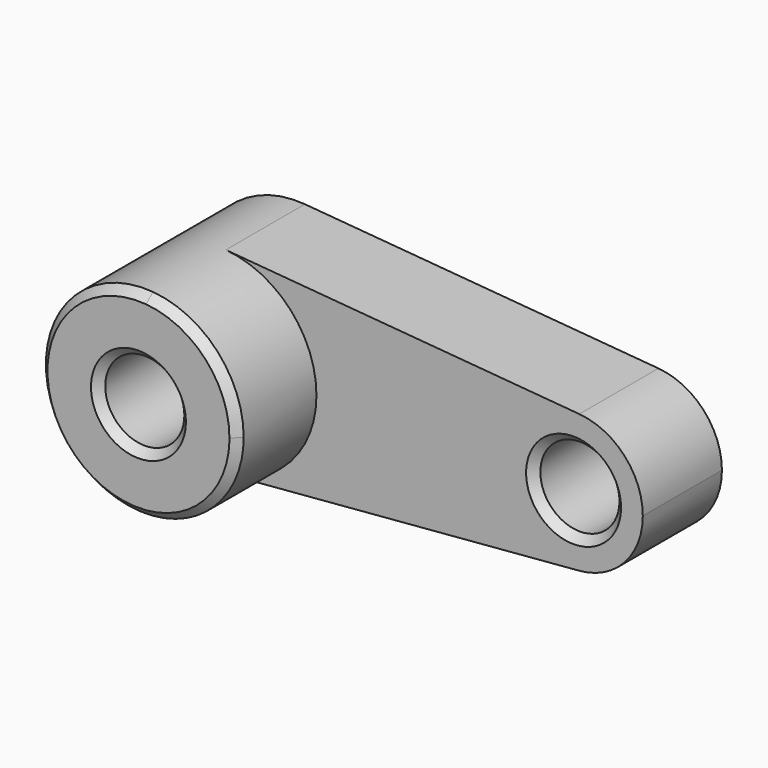
from build123d import *

# Parameters (mm, degrees)
F0_R     = 10
F1_DEPTH = 25
F2_DEPTH = 50
F3_SIZE  = 2


# Not quite as in the source:
# - the program builds the solid bodies; features that only make, move or delete a surface that nothing else refers to are left out


with BuildPart() as f1:
    # F0 (on Front) → F1 (new body)
    with BuildSketch(Plane.XZ):
        with BuildLine():
            ThreePointArc((2.0833333333, -24.9130432148), (18.3995018048, -16.9250800097), (25, 0))
            ThreePointArc((25, 0), (18.3995018048, 16.9250800097), (2.0833333333, 24.9130432148))
            ThreePointArc((2.0833333333, 24.9130432148), (-25, 0), (2.0833333333, -24.9130432148))
        make_face()
        Circle(F0_R, mode=Mode.SUBTRACT)
        with BuildLine():
            ThreePointArc((2.0833333333, 24.9130432148), (18.3995018048, 16.9250800097), (25, 0))
            ThreePointArc((25, 0), (18.3995018048, -16.9250800097), (2.0833333333, -24.9130432148))
            Line((2.0833333333, -24.9130432148), (91.4583333333, -17.4391302504))
            ThreePointArc((91.4583333333, -17.4391302504), (72.5, 0), (91.4583333333, 17.4391302504))
            Line((91.4583333333, 17.4391302504), (2.0833333333, 24.9130432148))
        make_face()
        with BuildLine():
            ThreePointArc((107.5, 0), (102.8796512634, 11.8475560068), (91.4583333333, 17.4391302504))
            ThreePointArc((91.4583333333, 17.4391302504), (72.5, 0), (91.4583333333, -17.4391302504))
            ThreePointArc((91.4583333333, -17.4391302504), (102.8796512634, -11.8475560068), (107.5, 0))
        make_face()
        with Locations((90, 0)):
            Circle(F0_R, mode=Mode.SUBTRACT)
    extrude(amount=F1_DEPTH)

    # F0 (on Front) → F2 (join)
    with BuildSketch(Plane.XZ):
        with BuildLine():
            ThreePointArc((2.0833333333, -24.9130432148), (18.3995018048, -16.9250800097), (25, 0))
            ThreePointArc((25, 0), (18.3995018048, 16.9250800097), (2.0833333333, 24.9130432148))
            ThreePointArc((2.0833333333, 24.9130432148), (-25, 0), (2.0833333333, -24.9130432148))
        make_face()
        Circle(F0_R, mode=Mode.SUBTRACT)
    extrude(amount=F2_DEPTH)

    # F3
    f3_edges = [f1.edges().sort_by_distance(p)[0] for p in [
        (-2.083333, -50, 24.913043),
        (-10, -50, 0),
        (80, -25, 0),
    ]]
    chamfer(f3_edges, length=F3_SIZE)


solid = f1.part
